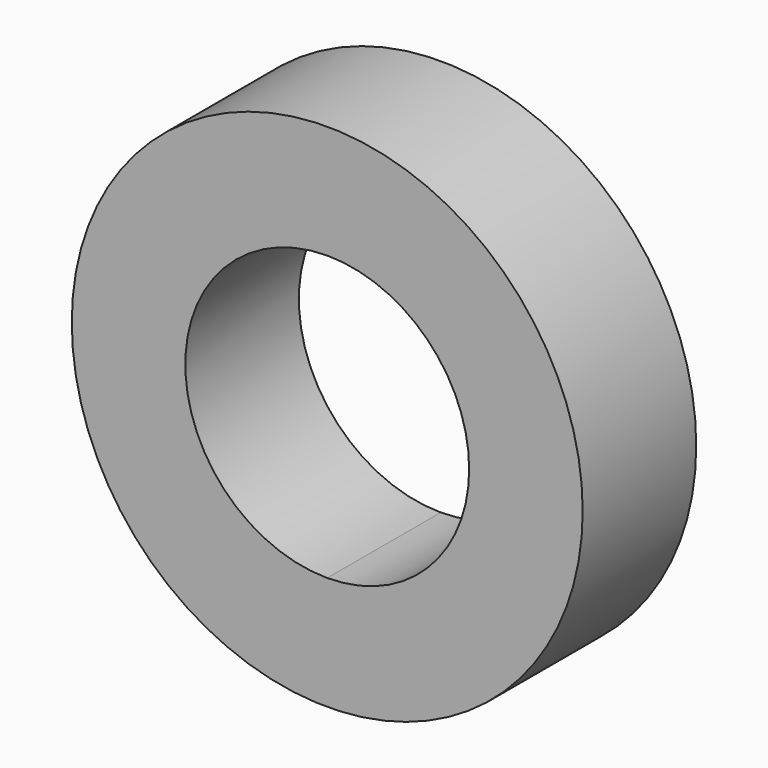
from build123d import *

# Parameters (mm, degrees)
F1_DEPTH = 25


with BuildPart() as f1:
    # F0 (on Front) → F1 (new body)
    with BuildSketch(Plane.XZ):
        with BuildLine():
            Line((0, 45), (45, 0))
            ThreePointArc((45, 0), (31.8198051534, 31.8198051534), (0, 45))
        make_face()
        with BuildLine():
            Line((0, -45), (45, 0))
            Line((45, 0), (0, 45))
            Line((0, 45), (0, 25))
            ThreePointArc((0, 25), (17.6776695297, 17.6776695297), (25, 0))
            ThreePointArc((25, 0), (17.6776695297, -17.6776695297), (0, -25))
            Line((0, -25), (0, -45))
        make_face()
        with BuildLine():
            ThreePointArc((0, -45), (31.8198051534, -31.8198051534), (45, 0))
            Line((45, 0), (0, -45))
        make_face()
        with BuildLine():
            Line((-45, 0), (0, 45))
            ThreePointArc((0, 45), (-31.8198051534, 31.8198051534), (-45, 0))
        make_face()
        with BuildLine():
            Line((0, 25), (0, 45))
            Line((0, 45), (-45, 0))
            Line((-45, 0), (0, -45))
            Line((0, -45), (0, -25))
            ThreePointArc((0, -25), (-25, 0), (0, 25))
        make_face()
        with BuildLine():
            ThreePointArc((-45, 0), (-31.8198051534, -31.8198051534), (0, -45))
            Line((0, -45), (-45, 0))
        make_face()
    extrude(amount=F1_DEPTH)


solid = f1.part
